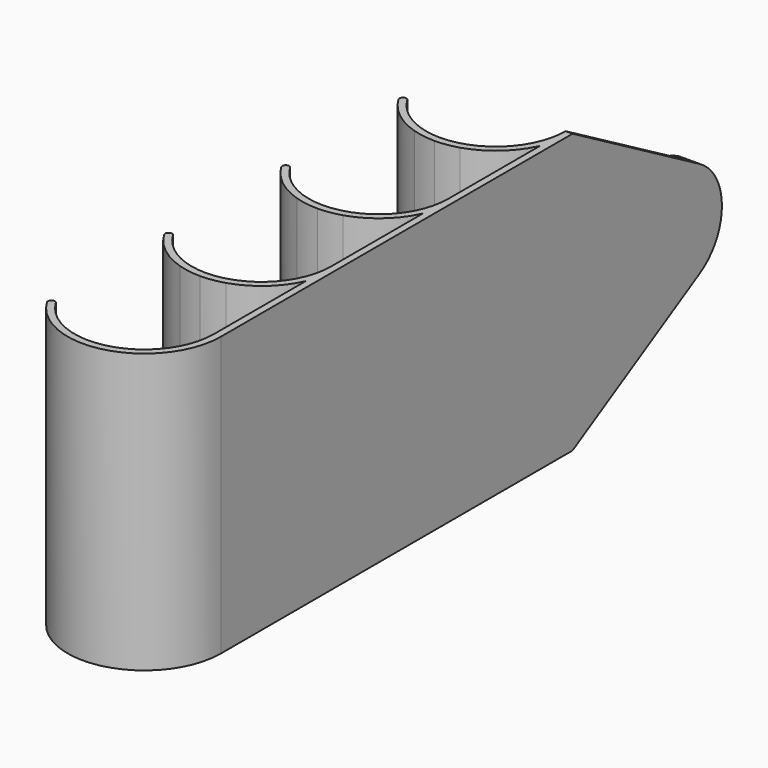
from build123d import *
from build123d import SkipClean  # not in build123d's __all__

# Parameters (mm, degrees)
F1_DEPTH = 40
F3_DEPTH = 1.001
F4_DEPTH = 2
F5_DEPTH = 0.5
F6_R     = 0.49999


# Not quite as in the source:
# - a fillet or chamfer is up to 0.001 mm smaller than in the source, because OpenCascade refuses the exact size


with BuildPart() as f1:
    # F0 (on Top) → F1 (new body)
    with BuildSketch(Plane.XY):
        with BuildLine():
            Line((11, 0), (10, 0))
            ThreePointArc((10, 0), (2.4380397486, -9.6982453147), (-8.8111924369, -4.7289415137))
            Line((-8.8111924369, -4.7289415137), (-9.6923116806, -5.2018356651))
            ThreePointArc((-9.6923116806, -5.2018356651), (2.6818437234, -10.6680698462), (11, 0))
        make_face()
        with BuildLine():
            Line((10, 4.582575695), (10, 0))
            Line((10, 0), (11, 0))
            ThreePointArc((11, 0), (10.7470926301, 2.3452078799), (10, 4.582575695))
        make_face()
        with BuildLine():
            Line((10, 16.417424305), (10, 4.582575695))
            ThreePointArc((10, 4.582575695), (10.7470926301, 2.3452078799), (11, 0))
            Line((11, 0), (11, 21))
            ThreePointArc((11, 21), (10.7470926301, 18.6547921201), (10, 16.417424305))
        make_face()
        with BuildLine():
            ThreePointArc((0, 11), (1.6583123952, 10.8742815855), (3.2787192622, 10.5))
            ThreePointArc((3.2787192622, 10.5), (7.2687738933, 12.743794692), (10, 16.417424305))
            Line((10, 16.417424305), (10, 21))
            ThreePointArc((10, 21), (7.0710678119, 13.9289321881), (0, 11))
        make_face()
        with BuildLine():
            ThreePointArc((-3.2787192622, 10.5), (-1.6583124171, 10.1257184179), (-4.44e-08, 10))
            ThreePointArc((-4.44e-08, 10), (1.6583123732, 10.1257184112), (3.2787192622, 10.5))
            ThreePointArc((3.2787192622, 10.5), (1.6583123952, 10.8742815855), (0, 11))
            ThreePointArc((0, 11), (-1.6583123952, 10.8742815855), (-3.2787192622, 10.5))
        make_face()
        with BuildLine():
            ThreePointArc((-9.6923116806, 15.7981643349), (-7.0056796429, 12.5194072884), (-3.2787192622, 10.5))
            ThreePointArc((-3.2787192622, 10.5), (-1.6583123952, 10.8742815855), (0, 11))
            ThreePointArc((0, 11), (-5.1337405886, 12.4183505333), (-8.8111924369, 16.2710584863))
            Line((-8.8111924369, 16.2710584863), (-9.6923116806, 15.7981643349))
        make_face()
        with BuildLine():
            Line((10, 21), (10, 16.417424305))
            ThreePointArc((10, 16.417424305), (10.7470926301, 18.6547921201), (11, 21))
            ThreePointArc((11, 21), (10.7470926301, 23.3452078799), (10, 25.582575695))
            Line((10, 25.582575695), (10, 21))
        make_face()
        with BuildLine():
            ThreePointArc((10, 25.582575695), (10.7470926301, 23.3452078799), (11, 21))
            Line((11, 21), (11, 42))
            ThreePointArc((11, 42), (10.7470926301, 39.6547921201), (10, 37.417424305))
            Line((10, 37.417424305), (10, 25.582575695))
        make_face()
        with BuildLine():
            ThreePointArc((5.81e-08, 32), (1.6583124239, 31.8742815811), (3.2787192622, 31.5))
            ThreePointArc((3.2787192622, 31.5), (7.2687738933, 33.743794692), (10, 37.417424305))
            Line((10, 37.417424305), (10, 42))
            ThreePointArc((10, 42), (7.0710678324, 34.9289322087), (5.81e-08, 32))
        make_face()
        with BuildLine():
            ThreePointArc((5.81e-08, 32), (-1.6583123665, 31.8742815898), (-3.2787192622, 31.5))
            ThreePointArc((-3.2787192622, 31.5), (-1.658312379, 31.1257184121), (3.28e-08, 31))
            ThreePointArc((3.28e-08, 31), (1.6583124114, 31.125718417), (3.2787192622, 31.5))
            ThreePointArc((3.2787192622, 31.5), (1.6583124239, 31.8742815811), (5.81e-08, 32))
        make_face()
        with BuildLine():
            ThreePointArc((-9.6923116806, 36.7981643349), (-7.0056796429, 33.5194072884), (-3.2787192622, 31.5))
            ThreePointArc((-3.2787192622, 31.5), (-1.6583123665, 31.8742815898), (5.81e-08, 32))
            ThreePointArc((5.81e-08, 32), (-5.1337405637, 33.4183505184), (-8.8111924369, 37.2710584863))
            Line((-8.8111924369, 37.2710584863), (-9.6923116806, 36.7981643349))
        make_face()
        with BuildLine():
            ThreePointArc((10, 37.417424305), (10.7470926301, 39.6547921201), (11, 42))
            ThreePointArc((11, 42), (10.7470926301, 44.3452078799), (10, 46.582575695))
            Line((10, 46.582575695), (10, 42))
            Line((10, 42), (10, 37.417424305))
        make_face()
        with BuildLine():
            ThreePointArc((10, 46.582575695), (10.7470926301, 44.3452078799), (11, 42))
            Line((11, 42), (11, 63))
            ThreePointArc((11, 63), (10.7470926301, 60.6547921201), (10, 58.417424305))
            Line((10, 58.417424305), (10, 46.582575695))
        make_face()
        with BuildLine():
            ThreePointArc((10, 58.417424305), (10.7470926301, 60.6547921201), (11, 63))
            ThreePointArc((11, 63), (10.8000300748, 65.0879057409), (10.2073908395, 67.0998990536))
            Line((10.2073908395, 67.0998990536), (10, 67.0998990536))
            Line((10, 67.0998990536), (10, 63))
            Line((10, 63), (10, 58.417424305))
        make_face()
        with BuildLine():
            ThreePointArc((0, 53), (1.6583123952, 52.8742815855), (3.2787192622, 52.5))
            ThreePointArc((3.2787192622, 52.5), (7.2687738933, 54.743794692), (10, 58.417424305))
            Line((10, 58.417424305), (10, 63))
            ThreePointArc((10, 63), (7.0710678119, 55.9289321881), (0, 53))
        make_face()
        with BuildLine():
            ThreePointArc((-5.66e-08, 52), (1.6583123672, 52.1257184103), (3.2787192622, 52.5))
            ThreePointArc((3.2787192622, 52.5), (1.6583123952, 52.8742815855), (0, 53))
            ThreePointArc((0, 53), (-1.6583123952, 52.8742815855), (-3.2787192622, 52.5))
            ThreePointArc((-3.2787192622, 52.5), (-1.6583124232, 52.1257184188), (-5.66e-08, 52))
        make_face()
        with BuildLine():
            ThreePointArc((-9.6923116806, 57.7981643349), (-7.0056796429, 54.5194072884), (-3.2787192622, 52.5))
            ThreePointArc((-3.2787192622, 52.5), (-1.6583123952, 52.8742815855), (0, 53))
            ThreePointArc((0, 53), (-5.1337405886, 54.4183505333), (-8.8111924369, 58.2710584863))
            Line((-8.8111924369, 58.2710584863), (-9.6923116806, 57.7981643349))
        make_face()
        with BuildLine():
            ThreePointArc((10, 67.582575695), (10.1065773297, 67.3424756395), (10.2073908395, 67.0998990536))
            Line((10.2073908395, 67.0998990536), (11, 67.0998990536))
            Line((11, 67.0998990536), (11, 89.784912765))
            Line((11, 89.784912765), (10, 89.784912765))
            Line((10, 89.784912765), (10, 67.582575695))
        make_face()
        with BuildLine():
            ThreePointArc((10.2073908395, 67.0998990536), (10.8000300748, 65.0879057409), (11, 63))
            Line((11, 63), (11, 67.0998990536))
            Line((11, 67.0998990536), (10.2073908395, 67.0998990536))
        make_face()
        with BuildLine():
            Line((10, 67.0998990536), (10.2073908395, 67.0998990536))
            ThreePointArc((10.2073908395, 67.0998990536), (10.1065773297, 67.3424756395), (10, 67.582575695))
            Line((10, 67.582575695), (10, 67.0998990536))
        make_face()
    extrude(amount=F1_DEPTH)

    # F2 (on face) → F3 (cut, through all)
    with BuildSketch(Plane(origin=(10, 0, 0), x_dir=(0, -1, 0), z_dir=(-1, 0, 0))):
        Polygon((-81.784912765, 10.7769520171), (-81.784912765, 0), (-63, 0), align=None)
        with BuildLine():
            Line((-89.784912765, 0), (-81.784912765, 0))
            Line((-81.784912765, 0), (-81.784912765, 10.7769520171))
            Line((-81.784912765, 10.7769520171), (-85.7659138368, 13.0608624119))
            ThreePointArc((-85.7659138368, 13.0608624119), (-88.7076293046, 15.9905117892), (-89.784912765, 20))
            Line((-89.784912765, 20), (-89.784912765, 0))
        make_face()
        with BuildLine():
            Line((-89.784912765, 40), (-89.784912765, 20))
            ThreePointArc((-89.784912765, 20), (-88.7076292465, 24.0094883112), (-85.7659136356, 26.9391377035))
            Line((-85.7659136356, 26.9391377035), (-81.784912765, 29.2230479829))
            Line((-81.784912765, 29.2230479829), (-81.784912765, 40))
            Line((-81.784912765, 40), (-89.784912765, 40))
        make_face()
        Polygon((-81.784912765, 29.2230479829), (-63, 40), (-81.784912765, 40), align=None)
    extrude(amount=-F3_DEPTH, mode=Mode.SUBTRACT)

    # F2 (on face) → F4 (join)
    with BuildSketch(Plane(origin=(10, 0, 0), x_dir=(0, -1, 0), z_dir=(-1, 0, 0))):
        with BuildLine():
            ThreePointArc((-85.7659138368, 13.0608624119), (-83.8448762714, 12.2697638877), (-81.784912765, 12))
            Line((-81.784912765, 12), (-81.784912765, 12.5))
            ThreePointArc((-81.784912765, 12.5), (-89.284912765, 20), (-81.784912765, 27.5))
            Line((-81.784912765, 27.5), (-81.784912765, 28))
            ThreePointArc((-81.784912765, 28), (-83.8448761593, 27.7302361422), (-85.7659136356, 26.9391377035))
            ThreePointArc((-85.7659136356, 26.9391377035), (-88.7076292465, 24.0094883112), (-89.784912765, 20))
            ThreePointArc((-89.784912765, 20), (-88.7076293046, 15.9905117892), (-85.7659138368, 13.0608624119))
        make_face()
        with BuildLine():
            Line((-81.784912765, 12.5), (-81.784912765, 12))
            ThreePointArc((-81.784912765, 12), (-76.1280585155, 14.3431457505), (-73.784912765, 20))
            ThreePointArc((-73.784912765, 20), (-76.1280585155, 25.6568542495), (-81.784912765, 28))
            Line((-81.784912765, 28), (-81.784912765, 27.5))
            ThreePointArc((-81.784912765, 27.5), (-76.4816119061, 25.3033008589), (-74.284912765, 20))
            ThreePointArc((-74.284912765, 20), (-76.4816119061, 14.6966991411), (-81.784912765, 12.5))
        make_face()
    with SkipClean():  # cleaning this boolean's faces spoils the solid; the shape is the same uncleaned
        extrude(amount=F4_DEPTH)

    # F2 (on face) → F5 (cut)
    with BuildSketch(Plane(origin=(10, 0, 0), x_dir=(0, -1, 0), z_dir=(-1, 0, 0))):
        with BuildLine():
            Line((-81.784912765, 27.5), (-81.784912765, 12.5))
            ThreePointArc((-81.784912765, 12.5), (-76.4816119061, 14.6966991411), (-74.284912765, 20))
            ThreePointArc((-74.284912765, 20), (-76.4816119061, 25.3033008589), (-81.784912765, 27.5))
        make_face()
        with BuildLine():
            ThreePointArc((-81.784912765, 27.5), (-89.284912765, 20), (-81.784912765, 12.5))
            Line((-81.784912765, 12.5), (-81.784912765, 27.5))
        make_face()
    with SkipClean():  # cleaning this boolean's faces spoils the solid; the shape is the same uncleaned
        extrude(amount=-F5_DEPTH, mode=Mode.SUBTRACT)

    # F6 (radius 0.5 in the source; OpenCascade refuses exactly that, so slightly less here)
    f6_edges = [f1.edges().sort_by_distance(p)[0] for p in [
        (-8.811192, 58.271058, 20),
        (-9.692312, 57.798164, 20),
        (-8.811192, 37.271058, 20),
        (-9.692312, 36.798164, 20),
        (-8.811192, 16.271058, 20),
        (-9.692312, 15.798164, 20),
        (-8.811192, -4.728942, 20),
        (-9.692312, -5.201836, 20),
    ]]
    fillet(f6_edges, radius=F6_R)


solid = f1.part
